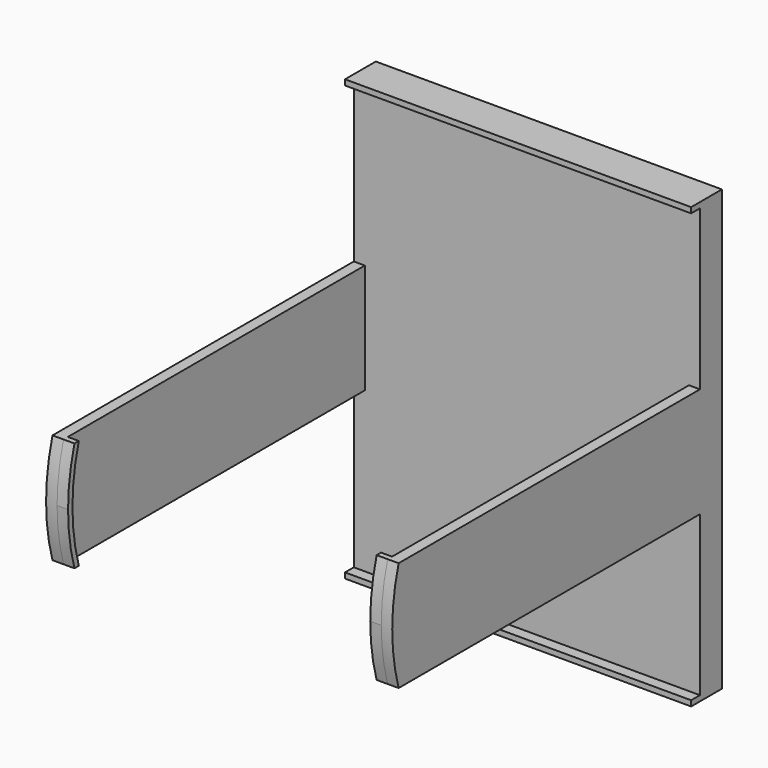
from build123d import *

# Parameters (mm, degrees)
F0_W      = 80
F0_H      = 101.6
F1_DEPTH  = 6.35
F3_DEPTH  = 2.54
F5_DEPTH  = 2.54
F7_DEPTH  = 2.54
F9_DEPTH  = 2.54
F10_W     = 80
F10_H     = 1.27
F11_DEPTH = 2.54
F12_DEPTH = 2.54


with BuildPart() as f1:
    # F0 (on Front) → F1 (new body)
    with BuildSketch(Plane.XZ):
        with Locations((18.1234987736, -29.8747005124)):
            Rectangle(F0_W, F0_H)
    extrude(amount=F1_DEPTH)

    # F2 (on face) → F3 (join)
    with BuildSketch(Plane.YZ.offset(58.1234987736)):
        with BuildLine():
            Line((-93.3970949714, -42.5747005124), (-6.35, -42.5747005124))
            Line((-6.35, -42.5747005124), (-6.35, -29.8747005124))
            Line((-6.35, -29.8747005124), (-6.35, -17.1747005124))
            Line((-6.35, -17.1747005124), (-93.3970949714, -17.1747005124))
            ThreePointArc((-93.3970949714, -17.1747005124), (-95.25, -29.8747005124), (-93.3970949714, -42.5747005124))
        make_face()
    extrude(amount=-F3_DEPTH)

    # F4 (on face) → F5 (join)
    with BuildSketch(Plane(origin=(-21.8765012264, 0, 0), x_dir=(0, -1, 0), z_dir=(-1, 0, 0))):
        with BuildLine():
            Line((93.3970949714, -17.1747005124), (6.35, -17.1747005124))
            Line((6.35, -17.1747005124), (6.35, -42.5747005124))
            Line((6.35, -42.5747005124), (93.3970949714, -42.5747005124))
            ThreePointArc((93.3970949714, -42.5747005124), (95.25, -29.8747005124), (93.3970949714, -17.1747005124))
        make_face()
    extrude(amount=-F5_DEPTH)

    # F6 (on face) → F7 (join)
    with BuildSketch(Plane.YZ.offset(-19.3365012264)):
        with BuildLine():
            ThreePointArc((-95.25, -29.8747005124), (-94.7843345492, -36.2919284389), (-93.3970949714, -42.5747005124))
            Line((-93.3970949714, -42.5747005124), (-92.1396846861, -42.5747005124))
            ThreePointArc((-92.1396846861, -42.5747005124), (-93.5175310216, -36.2910226765), (-93.98, -29.8747005124))
            Line((-93.98, -29.8747005124), (-95.25, -29.8747005124))
        make_face()
        with BuildLine():
            ThreePointArc((-93.3970949714, -17.1747005124), (-94.7843345492, -23.4574725858), (-95.25, -29.8747005124))
            Line((-95.25, -29.8747005124), (-93.98, -29.8747005124))
            ThreePointArc((-93.98, -29.8747005124), (-93.5175310216, -23.4583783483), (-92.1396846861, -17.1747005124))
            Line((-92.1396846861, -17.1747005124), (-93.3970949714, -17.1747005124))
        make_face()
    extrude(amount=F7_DEPTH)

    # F8 (on face) → F9 (join)
    with BuildSketch(Plane(origin=(55.5834987736, 0, 0), x_dir=(0, -1, 0), z_dir=(-1, 0, 0))):
        with BuildLine():
            Line((94.006845472, -29.8747005124), (95.25, -29.8747005124))
            ThreePointArc((95.25, -29.8747005124), (94.7843345492, -23.4574725858), (93.3970949714, -17.1747005124))
            Line((93.3970949714, -17.1747005124), (92.1270949714, -17.1747005124))
            ThreePointArc((92.1270949714, -17.1747005124), (93.5343618687, -23.4555210098), (94.006845472, -29.8747005124))
        make_face()
        with BuildLine():
            ThreePointArc((93.3970949714, -42.5747005124), (94.7843345492, -36.2919284389), (95.25, -29.8747005124))
            Line((95.25, -29.8747005124), (94.006845472, -29.8747005124))
            ThreePointArc((94.006845472, -29.8747005124), (93.5343618687, -36.293880015), (92.1270949714, -42.5747005124))
            Line((92.1270949714, -42.5747005124), (93.3970949714, -42.5747005124))
        make_face()
    extrude(amount=F9_DEPTH)

    # F10 (on face) → F11 (join)
    with BuildSketch(Plane.XZ.offset(6.35)):
        with Locations((18.1234987736, 20.2902994876)):
            Rectangle(F10_W, F10_H)
    extrude(amount=F11_DEPTH)

    # F10 (on face) → F12 (join)
    with BuildSketch(Plane.XZ.offset(6.35)):
        with Locations((18.1234987736, -80.0397005124)):
            Rectangle(F10_W, F10_H)
    extrude(amount=F12_DEPTH)


solid = f1.part
